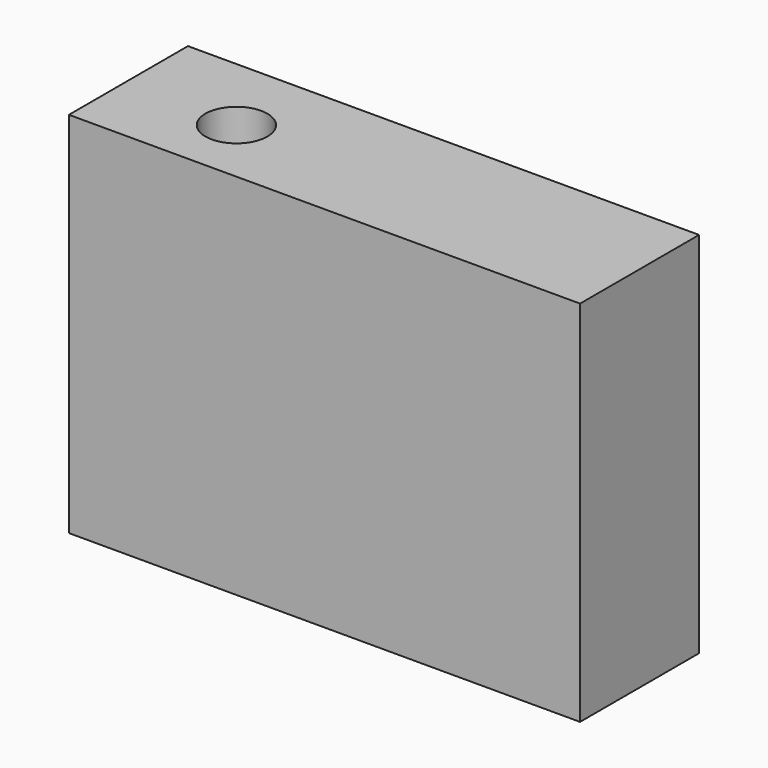
from build123d import *

# Parameters (mm, degrees)
F0_W     = 41.2274915725
F0_H     = 29.704278335
F2_DEPTH = 12
F5_D     = 5


# Not quite as in the source:
# - the program builds the solid bodies; features that only make, move or delete a surface that nothing else refers to are left out


with BuildPart() as f2:
    # F0 (on Front) → F2 (new body)
    with BuildSketch(Plane.XZ):
        with Locations((0.2560736611, -0.512146391)):
            Rectangle(F0_W, F0_H)
    extrude(amount=F2_DEPTH)

    # F5 (through all)
    with Locations(Plane.XY.offset(14.3399927765)):
        with Locations((-11.2421652302, -6.5094744787)):
            Hole(F5_D / 2)


solid = f2.part
